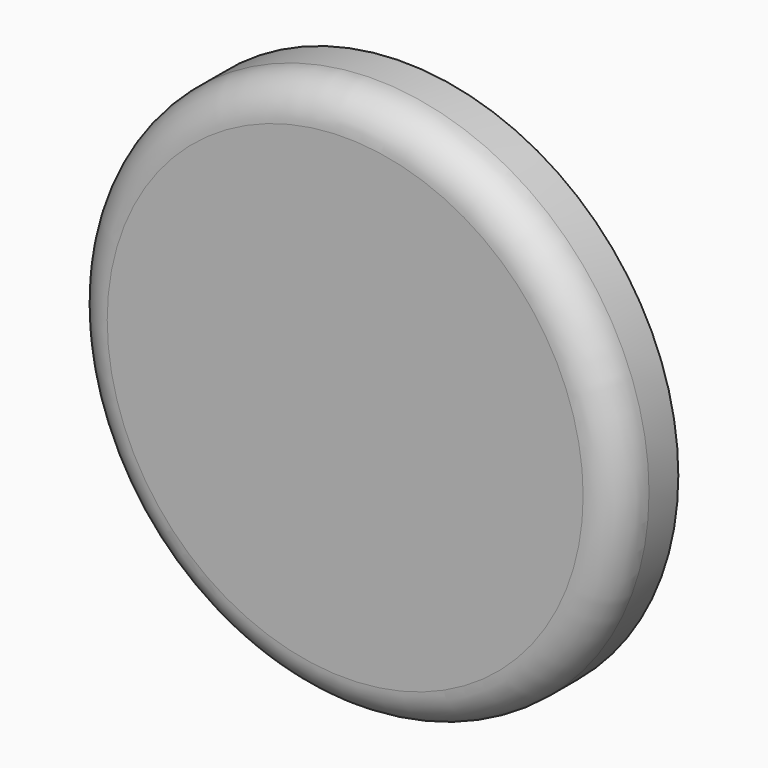
from build123d import *

# Parameters (mm, degrees)
F0_R          = 37.5
F1_DEPTH      = 5
F1_DEPTH_BACK = 5
F2_R          = 4.99999


# Not quite as in the source:
# - a fillet or chamfer is up to 0.001 mm smaller than in the source, because OpenCascade refuses the exact size


with BuildPart() as f1:
    # F0 (on Front) → F1 (new body, two sides)
    with BuildSketch(Plane.XZ) as f1_sk:
        Circle(F0_R)
    extrude(amount=F1_DEPTH)
    extrude(f1_sk.sketch, amount=-F1_DEPTH_BACK)

    # F2 (radius 5 in the source; OpenCascade refuses exactly that, so slightly less here)
    f2_edges = [f1.edges().sort_by_distance(p)[0] for p in [
        (-37.5, -5, 0),
    ]]
    fillet(f2_edges, radius=F2_R)


solid = f1.part
